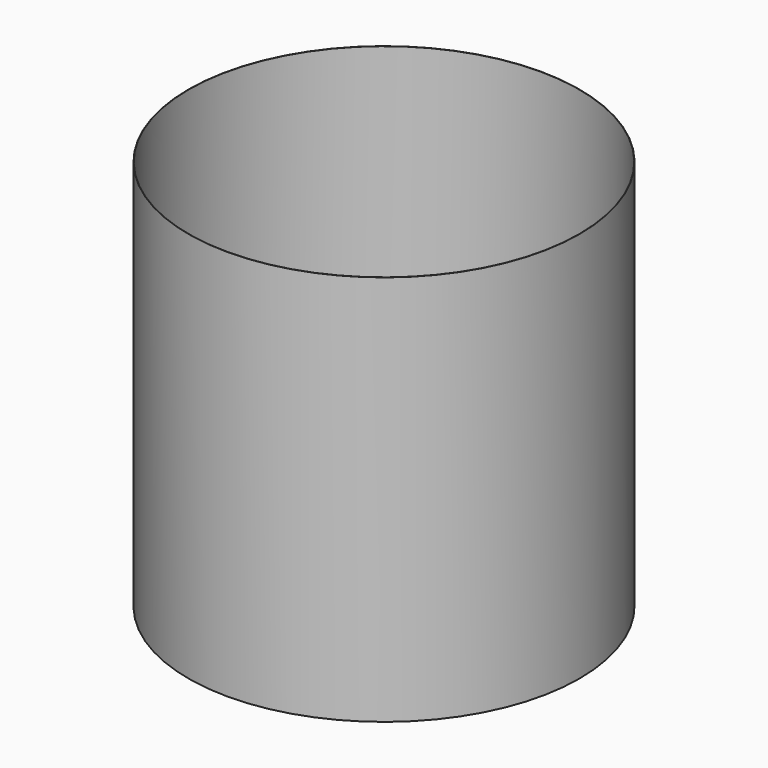
from build123d import *

# Parameters (mm, degrees)
F0_R     = 3048
F1_DEPTH = 6096
F2_T     = -3.048
F6_W     = 896.6910541058
F6_H     = 4.7625
F7_DEPTH = 1734.81703


# Not quite as in the source:
# - the program builds the solid bodies; features that only make, move or delete a surface that nothing else refers to are left out


with BuildPart() as f1:
    # F0 (on Top) → F1 (new body)
    with BuildSketch(Plane.XY):
        Circle(F0_R)
    extrude(amount=F1_DEPTH)

    # F2
    f2_openings = [f1.faces().sort_by_distance(p)[0] for p in [
        (0, 0, 6096),
    ]]
    offset(amount=F2_T, openings=f2_openings)

    # F6 (on Top) → F7 (cut)
    with BuildSketch(Plane.XY):
        with Locations((161.8346124887, -2.38125)):
            Rectangle(F6_W, F6_H)
    extrude(amount=F7_DEPTH, mode=Mode.SUBTRACT)


solid = f1.part
